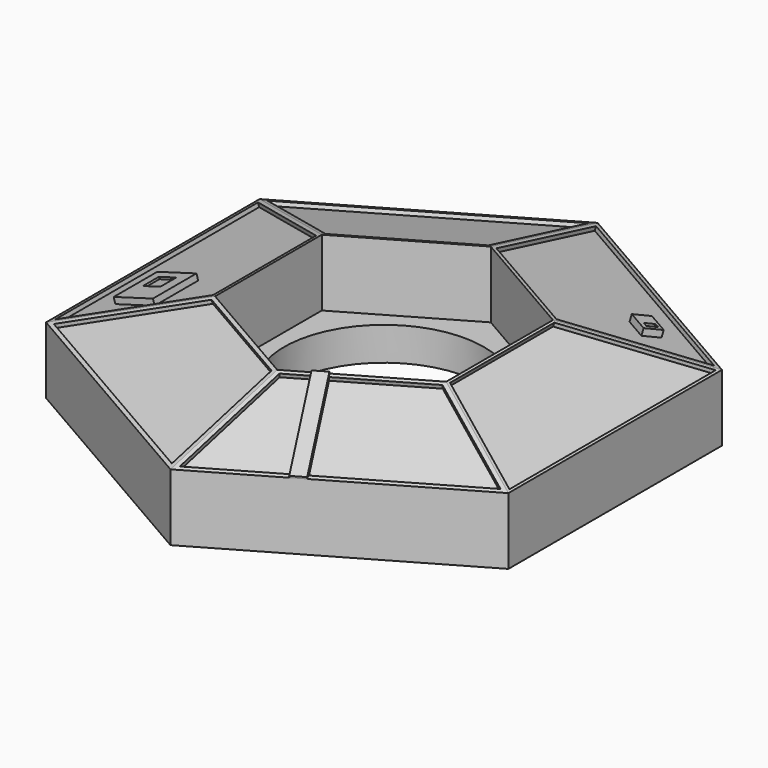
from build123d import *

# Parameters (mm, degrees)
F0_R      = 9.525
F1_DEPTH  = 6.35
F2_R      = 9.525
F3_DEPTH  = 3.175
F8_DEPTH  = 6.35
F9_W      = 3.8866475224
F9_H      = 5.1821961533
F9_W_2    = 1.7273994163
F9_H_2    = 1.9001385663
F10_DEPTH = 0.1905
F12_DEPTH = 0.1905
F13_DEPTH = 0.381
F15_DEPTH = 0.381
F17_DEPTH = 0.381
F18_W     = 3.8866475224
F18_H     = 5.1821961533
F19_DEPTH = 0.381
F21_DEPTH = 0.381
F23_DEPTH = 0.381
F25_DEPTH = 0.635


# Not quite as in the source:
# - a feature names something its author has since deleted; it is built from what else it names


with BuildPart() as f1:
    # F0 (on Top) → F1 (new body)
    with BuildSketch(Plane.XY):
        Polygon((21.9970452561, 12.7), (0, 25.4), (-21.9970452561, 12.7), (-21.9970452561, -12.7), (0, -25.4), (21.9970452561, -12.7), align=None)
        Polygon((-10.9985226281, 6.35), (0, 12.7), (10.9985226281, 6.35), (10.9985226281, -6.35), (0, -12.7), (-10.9985226281, -6.35), align=None, mode=Mode.SUBTRACT)
        Polygon((10.9985226281, 6.35), (0, 12.7), (-10.9985226281, 6.35), (-10.9985226281, -6.35), (0, -12.7), (10.9985226281, -6.35), align=None)
        Circle(F0_R, mode=Mode.SUBTRACT)
    extrude(amount=F1_DEPTH)

    # F2 (on face) → F3 (join)
    with BuildSketch(Plane.XY.offset(6.35)):
        Polygon((-10.9985226281, 6.35), (-10.9985226281, -6.35), (0, -12.7), (10.9985226281, -6.35), (10.9985226281, 6.35), (0, 12.7), align=None)
        Circle(F2_R, mode=Mode.SUBTRACT)
    extrude(amount=F3_DEPTH)

    # F4 (on face) → F6 section 0
    with BuildSketch(Plane.XY.offset(6.35)):
        Polygon((0, -25.4), (21.9970452561, -12.7), (21.9970452561, 12.7), (0, 25.4), (-21.9970452561, 12.7), (-21.9970452561, -12.7), align=None)
    # F5 (on face) → F6 section 1
    with BuildSketch(Plane.XY.offset(9.525)):
        Polygon((0, -12.7), (10.9985226281, -6.35), (10.9985226281, 6.35), (0, 12.7), (-10.9985226281, 6.35), (-10.9985226281, -6.35), align=None)
    loft()

    # F8 (cut): a face of the model
    f8_faces = [f1.faces().sort_by_distance(p)[0] for p in [
        (0, 0, 9.525),
    ]]
    extrude(f8_faces, amount=-F8_DEPTH, mode=Mode.SUBTRACT)

    # F9 (on face) → F10 (join)
    with BuildSketch(Plane(origin=(-3.3841608086, 0, 11.7230769231), x_dir=(0.9607689228, 0, 0.2773500981), z_dir=(-0.2773500981, 0, 0.9607689228))):
        with Locations((-14.8150864989, -5.1390115405)):
            Rectangle(F9_W, F9_H)
        with Locations((-14.9446423166, -4.4480519136)):
            Rectangle(F9_W_2, F9_H_2, mode=Mode.SUBTRACT)
    extrude(amount=F10_DEPTH)

    # F11 (on face) → F12 (join)
    with BuildSketch(Plane(origin=(1.6920804043, -2.9307692308, 11.7230769231), x_dir=(0.9903379377, 0.0336336397, -0.1345345588), z_dir=(0.1386750491, -0.2401922307, 0.9607689228))):
        Polygon((1.7312151801, -8.1025979269), (0.5512164028, -8.7571434803), (6.1041303172, -18.7678014037), (7.2841290946, -18.1132558503), align=None)
    extrude(amount=F12_DEPTH)

    # F7 (on face) → F13 (cut)
    with BuildSketch(Plane(origin=(3.3841608086, 0, 11.7230769231), x_dir=(0.9607689228, 0, -0.2773500981), z_dir=(0.2773500981, 0, 0.9607689228))):
        Polygon((8.1792790536, 6.2004337374), (8.1792790536, -6.2004337374), (19.1189043532, -12.2686460377), (19.1189043532, 12.2686460377), align=None)
    extrude(amount=-F13_DEPTH, mode=Mode.SUBTRACT)

    # F14 (on face) → F15 (cut)
    with BuildSketch(Plane(origin=(1.6920804043, 2.9307692308, 11.7230769231), x_dir=(0.9903379377, -0.0336336397, -0.1345345588), z_dir=(0.1386750491, 0.2401922307, 0.9607689228))):
        Polygon((-1.3275888968, 22.4544873413), (-1.3275888968, 10.2350073173), (9.3858632247, 4.2922533233), (19.7524424685, 10.7613898066), align=None)
    extrude(amount=-F15_DEPTH, mode=Mode.SUBTRACT)

    # F16 (on face) → F17 (cut)
    with BuildSketch(Plane(origin=(-1.6920804043, 2.9307692308, 11.7230769231), x_dir=(0.9903379377, 0.0336336397, 0.1345345588), z_dir=(-0.1386750491, 0.2401922307, 0.9607689228))):
        Polygon((-19.7524424685, 10.7613898066), (-9.3858632247, 4.2922533233), (1.3275888968, 10.2350073173), (1.3275888968, 22.4544873413), align=None)
    extrude(amount=-F17_DEPTH, mode=Mode.SUBTRACT)

    # F18 (on face) → F19 (cut)
    with BuildSketch(Plane(origin=(-3.3841608086, 0, 11.7230769231), x_dir=(0.9607689228, 0, 0.2773500981), z_dir=(-0.2773500981, 0, 0.9607689228))):
        Polygon((-8.3062790536, 6.1256506061), (-18.9919043532, 12.0529690566), (-18.9919043532, -12.0529690566), (-8.3062790536, -6.1256506061), align=None)
        with Locations((-14.8150864989, -5.1390115405)):
            Rectangle(F18_W, F18_H, mode=Mode.SUBTRACT)
    extrude(amount=-F19_DEPTH, mode=Mode.SUBTRACT)

    # F20 (on face) → F21 (cut)
    with BuildSketch(Plane(origin=(-1.6920804043, -2.9307692308, 11.7230769231), x_dir=(0.9903379377, -0.0336336397, 0.1345345588), z_dir=(-0.1386750491, -0.2401922307, 0.9607689228))):
        Polygon((1.3275888968, -22.4544873413), (1.3275888968, -10.2350073173), (-9.3858632247, -4.2922533233), (-19.7524424685, -10.7613898066), align=None)
    extrude(amount=-F21_DEPTH, mode=Mode.SUBTRACT)

    # F22 (on face) → F23 (cut)
    with BuildSketch(Plane(origin=(1.6920804043, -2.9307692308, 11.7230769231), x_dir=(0.9903379377, 0.0336336397, -0.1345345588), z_dir=(0.1386750491, -0.2401922307, 0.9607689228))):
        Polygon((9.3858632247, -4.2922533233), (1.9160273264, -8.4357727618), (7.0993169483, -17.7800810155), (19.7524424685, -10.7613898066), align=None)
        Polygon((5.9193181709, -18.4346265688), (0.736028549, -9.0903183152), (-1.3275888968, -10.2350073173), (-1.3275888968, -22.4544873413), align=None)
    extrude(amount=-F23_DEPTH, mode=Mode.SUBTRACT)

    # F24 (on face) → F25 (join)
    with BuildSketch(Plane(origin=(1.6392452106, 2.8392559909, 11.3570239635), x_dir=(0.9903379377, -0.0336336397, -0.1345345588), z_dir=(0.1386750491, 0.2401922307, 0.9607689228))):
        Polygon((14.1548511611, 11.4204940112), (12.0419776672, 12.5925053529), (11.9030368338, 12.3420262032), (11.2298887321, 11.1284912051), (13.3427622261, 9.9564798634), align=None)
        Polygon((12.6895471254, 10.7929574783), (13.1615737293, 11.6439155403), (13.6242877942, 11.3872479577), (13.1522611902, 10.5362898958), align=None, mode=Mode.SUBTRACT)
    extrude(amount=F25_DEPTH)


solid = f1.part
